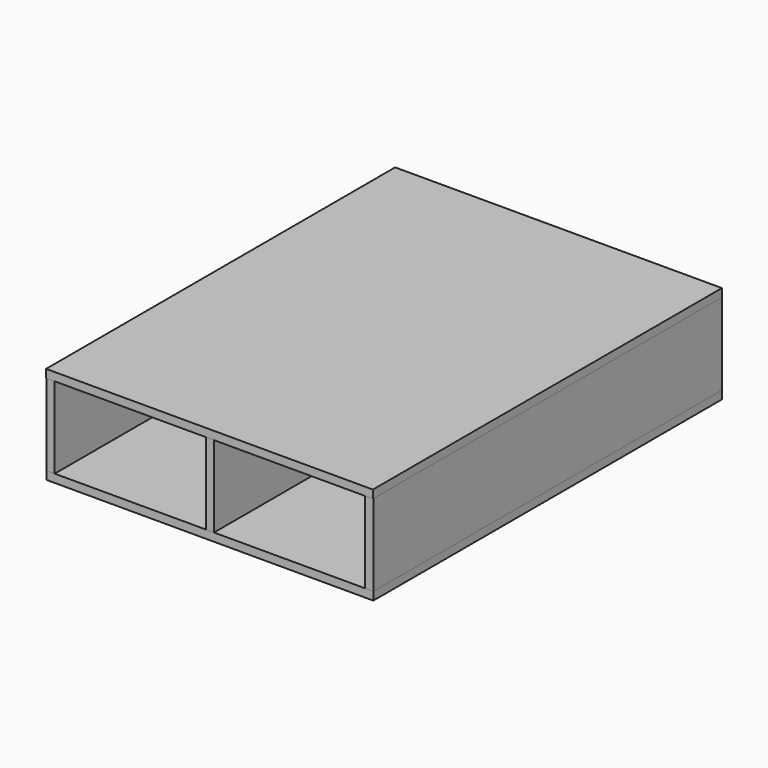
from build123d import *

# Parameters (mm, degrees)
F0_W     = 300
F0_H     = 400
F1_DEPTH = 15
F2_W     = 15
F2_H     = 800
F3_DEPTH = 150
F5_W     = 7.5
F5_H     = 800
F6_DEPTH = 150
F7_W     = 15
F7_H     = 800
F8_DEPTH = 15


with BuildPart() as f1:
    # F0 (on Top) → F1 (new body)
    with BuildSketch(Plane.XY):
        with Locations((-150, -200)):
            Rectangle(F0_W, F0_H)
        with Locations((150, -200)):
            Rectangle(F0_W, F0_H)
        with Locations((150, 200)):
            Rectangle(F0_W, F0_H)
        with Locations((-150, 200)):
            Rectangle(F0_W, F0_H)
    extrude(amount=F1_DEPTH)


with BuildPart() as f3:
    # F2 (on face) → F3 (new body)
    with BuildSketch(Plane.XY.offset(15)):
        with Locations((-292.5, 0)):
            Rectangle(F2_W, F2_H)
    extrude(amount=F3_DEPTH)


with BuildPart() as f4_1:
    # F4: instance of F3
    add(f3.part.mirror(Plane.YZ))


with BuildPart() as f6:
    # F5 (on face) → F6 (new body)
    with BuildSketch(Plane.XY.offset(15)):
        with Locations((3.75, 0)):
            Rectangle(F5_W, F5_H)
        with Locations((-3.75, 0)):
            Rectangle(F5_W, F5_H)
    extrude(amount=F6_DEPTH)


with BuildPart() as f8:
    # F7 (on face) → F8 (new body)
    with BuildSketch(Plane.XY.offset(165)):
        with Locations((-292.5, 0)):
            Rectangle(F7_W, F7_H)
        Polygon((300, 400), (-285, 400), (-285, -400), (-300, -400), (-300, -401.0900557041), (300, -401.0900557041), align=None)
    extrude(amount=F8_DEPTH)


solid = Compound([f1.part, f3.part, f4_1.part, f6.part, f8.part])
